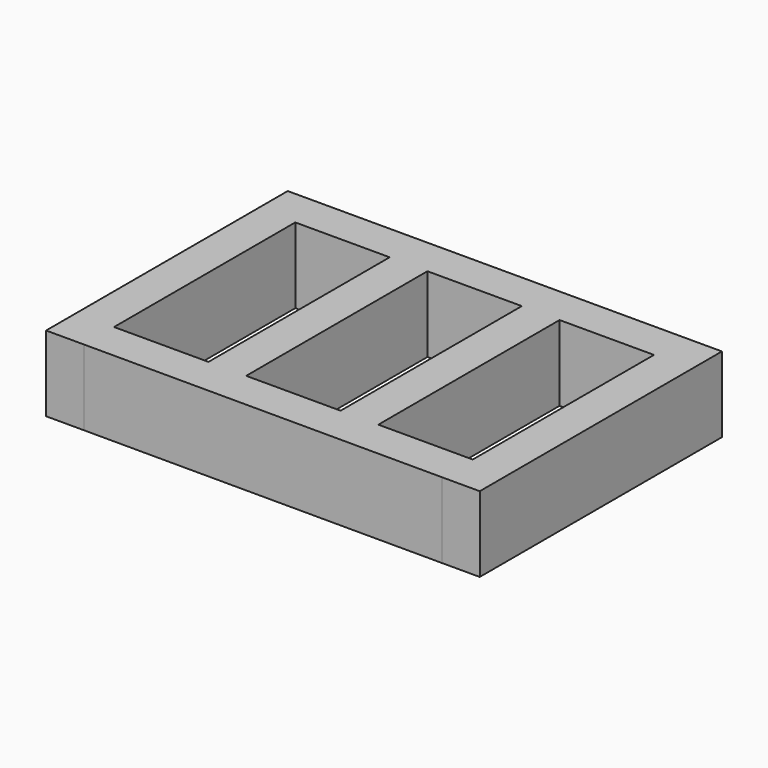
from build123d import *

# Parameters (mm, degrees)
F0_W     = 50.8
F0_H     = 304.8
F1_DEPTH = 101.6


# Not quite as in the source:
# - a feature names something its author has since deleted; it is built from what else it names


with BuildPart() as f1:
    # F0 (on Top) → F1 (new body)
    with BuildSketch(Plane.XY):
        Polygon((422.6718741447, 202.9749498913), (371.8718741447, 202.9749498913), (371.8718741447, 152.1749498913), (371.8718741447, -152.6250501087), (371.8718741447, -204.3104916811), (422.6718741447, -204.3104916811), align=None)
        Polygon((-110.7281258553, -152.6250501087), (-110.7281258553, 152.1749498913), (-110.7281258553, 202.9749498913), (-161.5281258553, 202.9749498913), (-161.5281258553, -152.6250501087), (-161.5281258553, -203.4250501087), (-110.7281258553, -203.4250501087), align=None)
        Polygon((-110.7281258553, 202.9749498913), (-110.7281258553, 152.1749498913), (16.2718741447, 152.1749498913), (67.0718741447, 152.1749498913), (194.0718741447, 152.1749498913), (244.8718741447, 152.1749498913), (371.8718741447, 152.1749498913), (371.8718741447, 202.9749498913), align=None)
        with Locations((41.6718741447, -0.2250501087)):
            Rectangle(F0_W, F0_H)
        with Locations((219.4718741447, -0.2250501087)):
            Rectangle(F0_W, F0_H)
        Polygon((16.2718741447, -152.6250501087), (-110.7281258553, -152.6250501087), (-110.7281258553, -203.4250501087), (371.8718741447, -204.3104916811), (371.8718741447, -152.6250501087), (244.8718741447, -152.6250501087), (194.0718741447, -152.6250501087), (67.0718741447, -152.6250501087), align=None)
    extrude(amount=F1_DEPTH)


solid = f1.part
